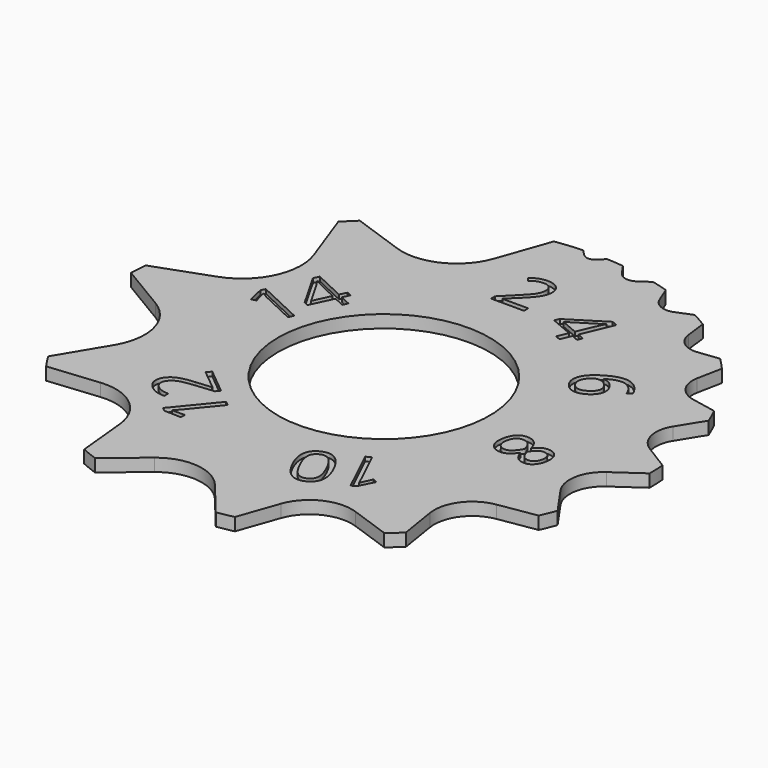
from build123d import *

# Parameters (mm, degrees)
F1_R         = 62.5
F2_DEPTH     = 3
F4_DEPTH     = 3.001
F5_D         = 50
F6_TEXT_SIZE = 16.6666666667
F7_DEPTH     = 1


# Not quite as in the source:
# - Text() gives the source's letters only with a copy of the font that has no kerning and outlines rounded to 1/6400 em; it was checked with that copy


with BuildPart() as f2:
    # F1 (on Top) → F2 (new body)
    with BuildSketch(Plane.XY):
        Circle(F1_R)
    extrude(amount=F2_DEPTH)

    # F3 (on Top) → F4 (cut, through all)
    with BuildSketch(Plane.XY):
        with BuildLine():
            Line((-2.8284271247, 62.4359671984), (-1.4142135624, 61.021753636))
            ThreePointArc((-1.4142135624, 61.021753636), (0, 60.4359671984), (1.4142135624, 61.021753636))
            Line((1.4142135624, 61.021753636), (2.8284271247, 62.4359671984))
            Line((2.8284271247, 62.4359671984), (0, 65.2643943231))
            Line((0, 65.2643943231), (-2.8284271247, 62.4359671984))
        make_face()
        with BuildLine():
            Line((6.8164899809, 62.1271717072), (8.530620265, 59.6651080669))
            ThreePointArc((8.530620265, 59.6651080669), (10.4638151573, 58.4262233075), (12.7068141895, 58.9171747107))
            Line((12.7068141895, 58.9171747107), (15.1688778298, 60.6313049949))
            Line((15.1688778298, 60.6313049949), (11.7406172615, 65.5554322755))
            Line((11.7406172615, 65.5554322755), (6.8164899809, 62.1271717072))
        make_face()
        with BuildLine():
            Line((19.0162282122, 59.5368210823), (20.520701129, 55.8305343634))
            ThreePointArc((20.520701129, 55.8305343634), (22.6700703776, 53.6504438066), (25.7314607647, 53.6287205613))
            Line((25.7314607647, 53.6287205613), (29.4377474836, 55.1331934781))
            Line((29.4377474836, 55.1331934781), (26.42880165, 62.5457669159))
            Line((26.42880165, 62.5457669159), (19.0162282122, 59.5368210823))
        make_face()
        with BuildLine():
            Line((32.9041762921, 53.1372297221), (33.4907168969, 48.1717518882))
            ThreePointArc((33.4907168969, 48.1717518882), (35.3598185217, 44.8324226057), (39.0427353356, 43.792814659))
            Line((39.0427353356, 43.792814659), (44.0082131695, 44.3793552638))
            Line((44.0082131695, 44.3793552638), (42.83513196, 54.3103109316))
            Line((42.83513196, 54.3103109316), (32.9041762921, 53.1372297221))
        make_face()
        with BuildLine():
            Line((46.7569084906, 41.4733831318), (45.5884412901, 35.5882591398))
            ThreePointArc((45.5884412901, 35.5882591398), (46.4859231182, 31.0846119375), (50.3050980816, 28.5346679473))
            Line((50.3050980816, 28.5346679473), (56.1902220736, 27.3662007468))
            Line((56.1902220736, 27.3662007468), (58.5271564746, 39.1364487309))
            Line((58.5271564746, 39.1364487309), (46.7569084906, 41.4733831318))
        make_face()
        with BuildLine():
            Line((57.8256843813, 23.7158222678), (54.1355656053, 17.7674591804))
            ThreePointArc((54.1355656053, 17.7674591804), (53.2684928067, 12.4805205383), (56.3938099166, 8.1289773171))
            Line((56.3938099166, 8.1289773171), (62.3421730039, 4.4388585411))
            Line((62.3421730039, 4.4388585411), (69.722410556, 16.3355847157))
            Line((69.722410556, 16.3355847157), (57.8256843813, 23.7158222678))
        make_face()
        with BuildLine():
            Line((62.4984376905, 0.4419120381), (55.9432982073, -4.1439517144))
            ThreePointArc((55.9432982073, -4.1439517144), (52.6512830226, -9.3066029743), (53.9740224765, -15.28495495))
            Line((53.9740224765, -15.28495495), (58.559886229, -21.8400944332))
            Line((58.559886229, -21.8400944332), (71.6701651954, -12.6683669283))
            Line((71.6701651954, -12.6683669283), (62.4984376905, 0.4419120381))
        make_face()
        with BuildLine():
            Line((57.0429053778, -25.5412792566), (48.1569025159, -26.9691984204))
            ThreePointArc((48.1569025159, -26.9691984204), (42.2917774747, -30.5815397247), (40.6988188178, -37.2831204461))
            Line((40.6988188178, -37.2831204461), (42.1267379816, -46.169123308))
            Line((42.1267379816, -46.169123308), (59.8987437054, -43.3132849804))
            Line((59.8987437054, -43.3132849804), (57.0429053778, -25.5412792566))
        make_face()
        with BuildLine():
            Line((39.0871517878, -48.7692994118), (29.6529946741, -45.4531752353))
            ThreePointArc((29.6529946741, -45.4531752353), (22.0107679202, -45.8715219867), (16.9027133839, -51.5712081725))
            Line((16.9027133839, -51.5712081725), (13.5865892074, -61.0053652862))
            Line((13.5865892074, -61.0053652862), (32.4549034349, -67.6376136392))
            Line((32.4549034349, -67.6376136392), (39.0871517878, -48.7692994118))
        make_face()
        with BuildLine():
            Line((9.6564200302, -61.749522688), (2.6631995585, -53.2586530368))
            ThreePointArc((2.6631995585, -53.2586530368), (-4.768672202, -49.3029683821), (-12.8208905644, -51.7610038573))
            Line((-12.8208905644, -51.7610038573), (-21.3117602156, -58.7542243291))
            Line((-21.3117602156, -58.7542243291), (-7.3253192722, -75.7359636315))
            Line((-7.3253192722, -75.7359636315), (9.6564200302, -61.749522688))
        make_face()
        with BuildLine():
            Line((-25.0264583362, -57.2706415465), (-26.2058076343, -45.3287348632))
            ThreePointArc((-26.2058076343, -45.3287348632), (-30.5374370075, -37.2299550791), (-39.3270636156, -34.5661774779))
            Line((-39.3270636156, -34.5661774779), (-51.2689702989, -35.7455267759))
            Line((-51.2689702989, -35.7455267759), (-48.9102717029, -59.6293401425))
            Line((-48.9102717029, -59.6293401425), (-25.0264583362, -57.2706415465))
        make_face()
        with BuildLine():
            Line((-53.450513552, -32.3927862498), (-46.7764817271, -21.2367430803))
            ThreePointArc((-46.7764817271, -21.2367430803), (-45.3247579589, -11.3934506403), (-51.2584930716, -3.4066680859))
            Line((-51.2584930716, -3.4066680859), (-62.4145362411, 3.267363739))
            Line((-62.4145362411, 3.267363739), (-75.762599891, -19.0447226))
            Line((-75.762599891, -19.0447226), (-53.450513552, -32.3927862498))
        make_face()
        with BuildLine():
            Line((-62.077707084, 7.2531567742), (-48.9109510803, 12.0109436902))
            ThreePointArc((-48.9109510803, 12.0109436902), (-40.9941721481, 19.2316606293), (-40.5019819926, 29.93548661))
            Line((-40.5019819926, 29.93548661), (-45.2597689087, 43.1022426137))
            Line((-45.2597689087, 43.1022426137), (-71.5932809161, 33.5866687816))
            Line((-71.5932809161, 33.5866687816), (-62.077707084, 7.2531567742))
        make_face()
        with BuildLine():
            Line((-42.4099461107, 45.909110979), (-30.1462294399, 41.5961939362))
            ThreePointArc((-30.1462294399, 41.5961939362), (-20.2112480643, 42.1384604988), (-13.5695957263, 49.5469935642))
            Line((-13.5695957263, 49.5469935642), (-9.2566786835, 61.810710235))
            Line((-9.2566786835, 61.810710235), (-33.7841120251, 70.4365443206))
            Line((-33.7841120251, 70.4365443206), (-42.4099461107, 45.909110979))
        make_face()
    extrude(amount=F4_DEPTH, mode=Mode.SUBTRACT)

    # F5 (through all)
    with Locations(Plane(origin=(0, 0, 0), x_dir=(1, 0, 0), z_dir=(0, 0, -1))):
        with Locations((0, 0)):
            Hole(F5_D / 2)

    # F6 (on face) → F7 (cut)
    with BuildSketch(Plane.XY.offset(3)):
        with Locations((-4.8580729167, 36.7179835992)):
            Text('2', F6_TEXT_SIZE, font='Open Sans', text_align=(TextAlign.LEFT, TextAlign.BOTTOM))
        with Locations(Location((9.1321851059, 34.8125061474), (0, 0, -22.9065569005))):
            Text('4', F6_TEXT_SIZE, font='Open Sans', text_align=(TextAlign.LEFT, TextAlign.BOTTOM))
        with Locations(Location((25.9233787717, 23.2273598728), (0, 0, -56.229800336))):
            Text('6', F6_TEXT_SIZE, font='Open Sans', text_align=(TextAlign.LEFT, TextAlign.BOTTOM))
        with Locations(Location((33.5747390168, -0.9853978981), (0, 0, -100.0240203747))):
            Text('8', F6_TEXT_SIZE, font='Open Sans', text_align=(TextAlign.LEFT, TextAlign.BOTTOM))
        with Locations(Location((22.5220685829, -24.6192082221), (0, 0, -154.3666719288))):
            Text('10', F6_TEXT_SIZE, font='Open Sans', text_align=(TextAlign.LEFT, TextAlign.BOTTOM))
        with Locations(Location((-11.9511328283, -29.7430558489), (0, 0, 140.6400824726))):
            Text('12', F6_TEXT_SIZE, font='Open Sans', text_align=(TextAlign.LEFT, TextAlign.BOTTOM))
        with Locations(Location((-30.5874004157, 3.4116407438), (0, 0, 64.8672434351))):
            Text('14', F6_TEXT_SIZE, font='Open Sans', text_align=(TextAlign.LEFT, TextAlign.BOTTOM))
    extrude(amount=-F7_DEPTH, mode=Mode.SUBTRACT)


solid = f2.part
